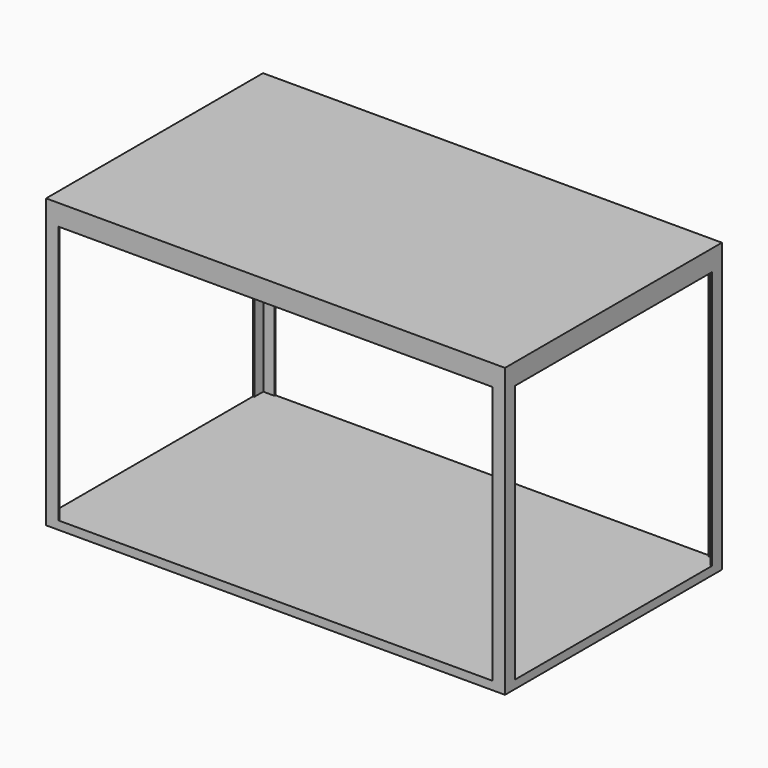
from build123d import *

# Parameters (mm, degrees)
F0_W           = 1100
F0_H           = 650
F1_DEPTH       = 20
F3_W           = 1100
F3_H           = 650
F4_DEPTH       = 20
F6_DEPTH       = 650
F10_DEPTH      = 322
F10_DEPTH_BACK = 322
F13_DEPTH      = 550
F13_DEPTH_BACK = 550


with BuildPart() as f1:
    # F0 (on Top) → F1 (new body)
    with BuildSketch(Plane.XY):
        Rectangle(F0_W, F0_H)
    extrude(amount=-F1_DEPTH)



with BuildPart() as f4:
    # F3 (on offset) → F4 (new body)
    with BuildSketch(Plane.XY.offset(650)):
        Rectangle(F3_W, F3_H)
    extrude(amount=F4_DEPTH)


with BuildPart() as f1_1:
    add(f1.part)

    add(f4.part)  # F6 merges F4
    # F5 (on face) → F6 (join, through all)
    with BuildSketch(Plane.XY):
        Polygon((-547, -295), (-550, -295), (-550, -325), (-520, -325), (-520, -322), (-547, -322), align=None)
    extrude(amount=F6_DEPTH)

    # F7: F1 across plane


with BuildPart() as f1_2:
    add(f1_1.part)
    add(f1_1.part.mirror(Plane.XZ))

    # F8: F1 across plane


with BuildPart() as f1_3:
    add(f1_2.part)
    add(f1_2.part.mirror(Plane.YZ))

    # F9 (on Front) → F10 (join, two sides)
    with BuildSketch(Plane.XZ) as f10_sk:
        Polygon((-520, 647), (-520, 650), (-550, 650), (-550, 620), (-547, 620), (-547, 647), align=None)
    extrude(amount=F10_DEPTH)
    extrude(f10_sk.sketch, amount=-F10_DEPTH_BACK)

    # F11: F1 across plane


with BuildPart() as f1_4:
    add(f1_3.part)
    add(f1_3.part.mirror(Plane.YZ))

    # F12 (on Right) → F13 (join, two sides)
    with BuildSketch(Plane.YZ) as f13_sk:
        Polygon((-295, 650), (-325, 650), (-325, 620), (-322, 620), (-322, 647), (-295, 647), align=None)
    extrude(amount=F13_DEPTH)
    extrude(f13_sk.sketch, amount=-F13_DEPTH_BACK)

    # F14: F1 across plane


with BuildPart() as f1_5:
    add(f1_4.part)
    add(f1_4.part.mirror(Plane.XZ))


solid = f1_5.part
